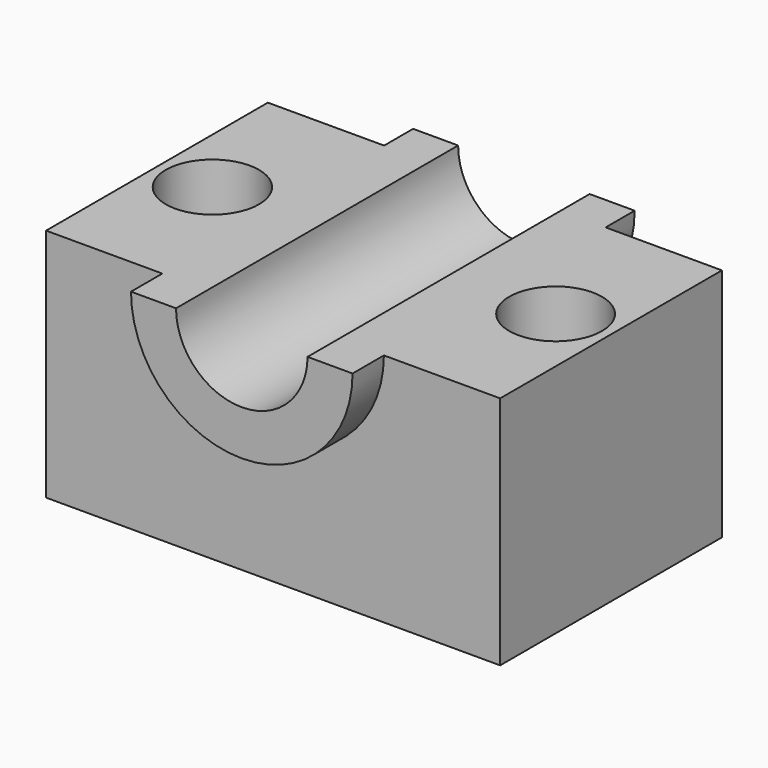
from build123d import *

# Parameters (mm, degrees)
F0_W     = 147.184163332
F0_H     = 89.8508056998
F0_R     = 15.1184260195
F0_R_2   = 15.0482996588
F1_DEPTH = 76.2
F3_DEPTH = 101.6
F4_DEPTH = 12.7
F6_DEPTH = 114.301


with BuildPart() as f1:
    # F0 (on Top) → F1 (new body)
    with BuildSketch(Plane.XY):
        Rectangle(F0_W, F0_H)
        with Locations((-55.6219257414, 0)):
            Circle(F0_R, mode=Mode.SUBTRACT)
        with Locations((55.6219220161, 0)):
            Circle(F0_R_2, mode=Mode.SUBTRACT)
    extrude(amount=F1_DEPTH)

    # F2 (on face) → F3 (join)
    with BuildSketch(Plane.XZ.offset(44.9254028499)):
        with BuildLine():
            ThreePointArc((-35.903516253, 76.2), (0, 40.296483747), (35.903516253, 76.2))
            Line((35.903516253, 76.2), (-35.903516253, 76.2))
        make_face()
    extrude(amount=-F3_DEPTH)

    # F2 (on face) → F4 (join)
    with BuildSketch(Plane.XZ.offset(44.9254028499)):
        with BuildLine():
            ThreePointArc((-35.903516253, 76.2), (0, 40.296483747), (35.903516253, 76.2))
            Line((35.903516253, 76.2), (-35.903516253, 76.2))
        make_face()
    extrude(amount=F4_DEPTH)

    # F5 (on face) → F6 (cut, through all)
    with BuildSketch(Plane.XZ.offset(57.6254028499)):
        with BuildLine():
            Line((-21.3098982127, 76.2), (21.3098982127, 76.2))
            ThreePointArc((21.3098982127, 76.2), (0, 97.5098982127), (-21.3098982127, 76.2))
        make_face()
        with BuildLine():
            ThreePointArc((-21.3098982127, 76.2), (0, 54.8901017873), (21.3098982127, 76.2))
            Line((21.3098982127, 76.2), (-21.3098982127, 76.2))
        make_face()
    extrude(amount=-F6_DEPTH, mode=Mode.SUBTRACT)


solid = f1.part
